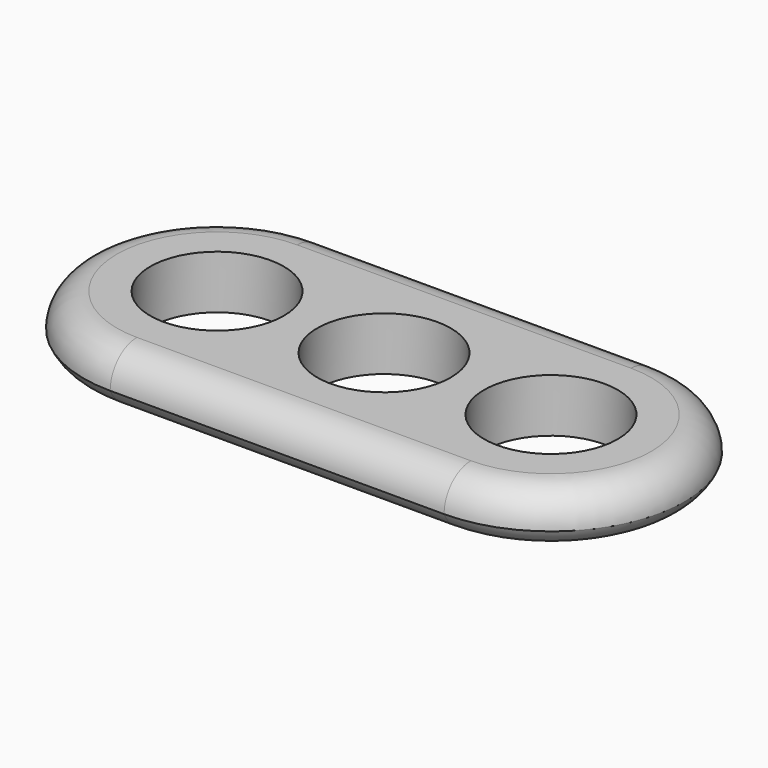
from build123d import *

# Parameters (mm, degrees)
F0_R        = 10
F1_DEPTH    = 4
F2_R        = 5
F3_T1_DEPTH = 50
F3_T4_ANGLE = 180
F3_T6_ANGLE = 180


# Not quite as in the source:
# - a fillet or chamfer that OpenCascade refuses, or shapes differently, is made with other operations: its cross-section is extruded or revolved along the edge and cut away or added


with BuildPart() as f1:
    # F0 (on Top) → F1 (new body, symmetric)
    with BuildSketch(Plane.XY):
        with BuildLine():
            Line((25, 20), (-25, 20))
            ThreePointArc((-25, 20), (-45, 0), (-25, -20))
            Line((-25, -20), (25, -20))
            ThreePointArc((25, -20), (45, 0), (25, 20))
        make_face()
        with Locations((-25, 0)):
            Circle(F0_R, mode=Mode.SUBTRACT)
        Circle(F0_R, mode=Mode.SUBTRACT)
        with Locations((25, 0)):
            Circle(F0_R, mode=Mode.SUBTRACT)
    extrude(amount=F1_DEPTH, both=True)

    # F2
    f2_edges = [f1.edges().sort_by_distance(p)[0] for p in [
        (0, 20, 4),
        (-45, 0, 4),
        (0, -20, 4),
        (45, 0, 4),
    ]]
    fillet(f2_edges, radius=F2_R)

    # F3: fillet of radius 5 on 4 edges, made by hand

    # F3_s2 → F3_t1 (cut)
    with BuildSketch(Plane.YZ.offset(-25)):
        with BuildLine():
            ThreePointArc((-15.417424305, -4), (-18.1560370926, -3.1833001327), (-20, -1))
            Line((-20, -1), (-20, -4))
            Line((-20, -4), (-15.417424305, -4))
        make_face()
        with BuildLine():
            ThreePointArc((20, -1), (18.1560370926, -3.1833001327), (15.417424305, -4))
            Line((15.417424305, -4), (20, -4))
            Line((20, -4), (20, -1))
        make_face()
    extrude(amount=F3_T1_DEPTH, mode=Mode.SUBTRACT)

    # F3_s3 → F3_t4 (revolve, cut)
    with BuildSketch(Plane.YZ.offset(25)):
        with BuildLine():
            ThreePointArc((-20, -1), (-18.1560370926, -3.1833001327), (-15.417424305, -4))
            Line((-15.417424305, -4), (-20, -4))
            Line((-20, -4), (-20, -1))
        make_face()
    revolve(axis=Axis((25, 0, -4), (0, 0, 1)), revolution_arc=F3_T4_ANGLE, mode=Mode.SUBTRACT)

    # F3_s5 → F3_t6 (revolve, cut)
    with BuildSketch(Plane.YZ.offset(-25)):
        with BuildLine():
            ThreePointArc((15.417424305, -4), (18.1560370926, -3.1833001327), (20, -1))
            Line((20, -1), (20, -4))
            Line((20, -4), (15.417424305, -4))
        make_face()
    revolve(axis=Axis((-25, 0, -4), (0, 0, 1)), revolution_arc=F3_T6_ANGLE, mode=Mode.SUBTRACT)


solid = f1.part
